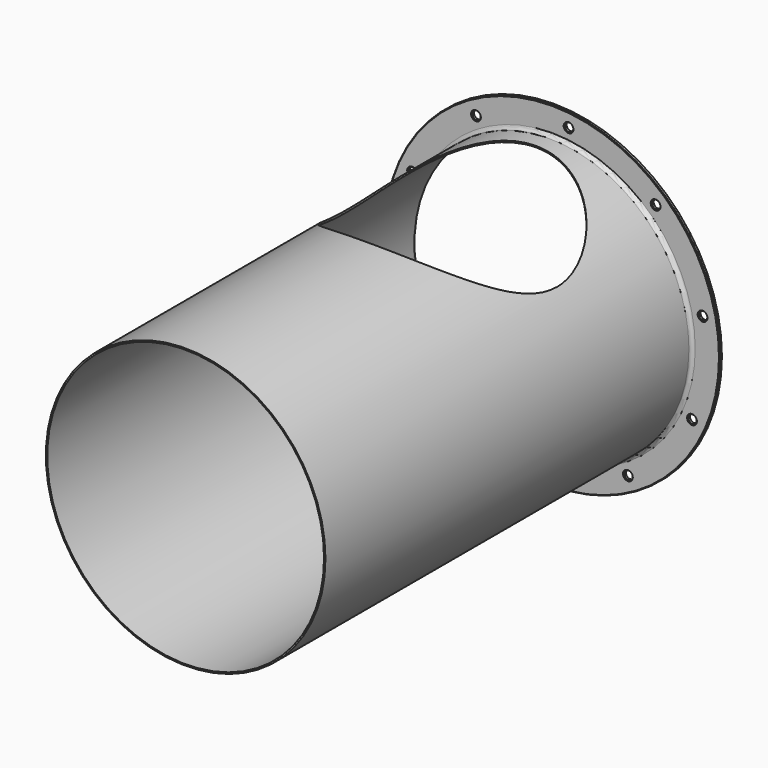
from build123d import *

# Parameters (mm, degrees)
F0_R     = 200
F0_R_2   = 198
F1_DEPTH = 655
F0_R_3   = 240
F0_R_4   = 6
F2_DEPTH = 5
F4_R     = 5
F5_SIZE  = 1
F6_SIZE  = 1
F8_D     = 300
F8_DEPTH = 240.001


# Not quite as in the source:
# - a fillet or chamfer that OpenCascade refuses, or shapes differently, is made with other operations: its cross-section is extruded or revolved along the edge and cut away or added
# - a feature names something its author has since deleted; it is built from what else it names


with BuildPart() as f1:
    # F0 (on Front) → F1 (new body)
    with BuildSketch(Plane.XZ):
        Circle(F0_R)
        Circle(F0_R_2, mode=Mode.SUBTRACT)
    extrude(amount=F1_DEPTH)

    # F0 (on Front) → F2 (join)
    with BuildSketch(Plane.XZ):
        Circle(F0_R_3)
        with Locations((-148.3494010818, -162.4575489125)):
            Circle(F0_R_4, mode=Mode.SUBTRACT)
        with Locations((-24.5270352061, -218.6285080771)):
            Circle(F0_R_4, mode=Mode.SUBTRACT)
        with Locations((-215.5073379549, -44.2333277925)):
            Circle(F0_R_4, mode=Mode.SUBTRACT)
        with Locations((108.663824475, -191.2908080658)):
            Circle(F0_R_4, mode=Mode.SUBTRACT)
        with Locations((200.3487965542, -90.8865211088)):
            Circle(F0_R_4, mode=Mode.SUBTRACT)
        with Locations((-200.0304758549, 90.5413627625)):
            Circle(F0_R_4, mode=Mode.SUBTRACT)
        with Locations((-108.663824475, 191.2908080658)):
            Circle(F0_R_4, mode=Mode.SUBTRACT)
        Circle(F0_R, mode=Mode.SUBTRACT)
        with Locations((215.5073379549, 44.2333277925)):
            Circle(F0_R_4, mode=Mode.SUBTRACT)
        with Locations((23.8151364028, 219.3368971348)):
            Circle(F0_R_4, mode=Mode.SUBTRACT)
        with Locations((148.3494010818, 162.4575489125)):
            Circle(F0_R_4, mode=Mode.SUBTRACT)
        Circle(F0_R)
        Circle(F0_R_2, mode=Mode.SUBTRACT)
    extrude(amount=-F2_DEPTH)

    # F3: fillet of radius 5 on 1 edges, made by hand

    # F3_s1 → F3_t2 (revolve, cut)
    with BuildSketch(Plane.XY):
        with BuildLine():
            ThreePointArc((198, 0), (199.4644660941, 3.5355339059), (203, 5))
            Line((203, 5), (198, 5))
            Line((198, 5), (198, 0))
        make_face()
    revolve(axis=Axis((0, 5, 0), (0, -1, 0)), mode=Mode.SUBTRACT)

    # F4
    f4_edges = [f1.edges().sort_by_distance(p)[0] for p in [
        (-200, 0, 0),
    ]]
    fillet(f4_edges, radius=F4_R)

    # F5
    f5_edges = [f1.edges().sort_by_distance(p)[0] for p in [
        (-205, 0, 0),
        (-240, 0, 0),
        (-154.349401, 0, -162.457549),
        (-30.527035, 0, -218.628508),
        (-221.507338, 0, -44.233328),
        (102.663824, 0, -191.290808),
        (194.348797, 0, -90.886521),
        (-206.030476, 0, 90.541363),
        (-114.663824, 0, 191.290808),
        (209.507338, 0, 44.233328),
        (17.815136, 0, 219.336897),
        (142.349401, 0, 162.457549),
    ]]
    chamfer(f5_edges, length=F5_SIZE)

    # F6
    f6_edges = [f1.edges().sort_by_distance(p)[0] for p in [
        (-240, 5, 0),
        (-154.349401, 5, -162.457549),
        (-30.527035, 5, -218.628508),
        (-221.507338, 5, -44.233328),
        (102.663824, 5, -191.290808),
        (-203, 5, 0),
        (194.348797, 5, -90.886521),
        (-206.030476, 5, 90.541363),
        (-114.663824, 5, 191.290808),
        (209.507338, 5, 44.233328),
        (17.815136, 5, 219.336897),
        (142.349401, 5, 162.457549),
    ]]
    chamfer(f6_edges, length=F6_SIZE)

    # F8 (through all, one way)
    with BuildSketch(Plane(origin=(0, 0, 0), x_dir=(1, 0, 0), z_dir=(0, 0, -1))):
        with Locations((0, 178.1619042158)):
            Circle(F8_D / 2)
    extrude(amount=-F8_DEPTH, mode=Mode.SUBTRACT)


solid = f1.part
